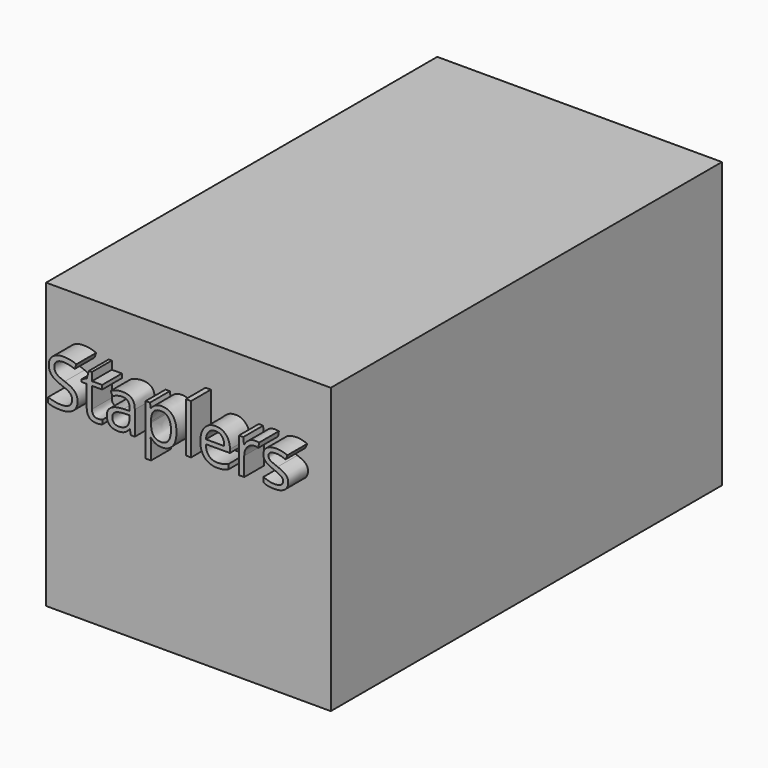
from build123d import *

# Parameters (mm, degrees)
F0_W         = 292.1
F0_H         = 292.1
F1_DEPTH     = 501.65
F2_TEXT_SIZE = 67.0350515464
F3_DEPTH     = 25.4


# Not quite as in the source:
# - Text() gives the source's letters only with a copy of the font that has no kerning and outlines rounded to 1/6400 em; it was checked with that copy


with BuildPart() as f1:
    # F0 (on Front) → F1 (new body)
    with BuildSketch(Plane.XZ):
        Rectangle(F0_W, F0_H)
    extrude(amount=F1_DEPTH)

    # F2 (on face) → F3 (join)
    with BuildSketch(Plane.XZ.offset(501.65)):
        with Locations((-127, 53.4118779413)):
            Text('Staplers', F2_TEXT_SIZE, font='Open Sans', text_align=(TextAlign.LEFT, TextAlign.BOTTOM))
    extrude(amount=F3_DEPTH)


solid = f1.part
